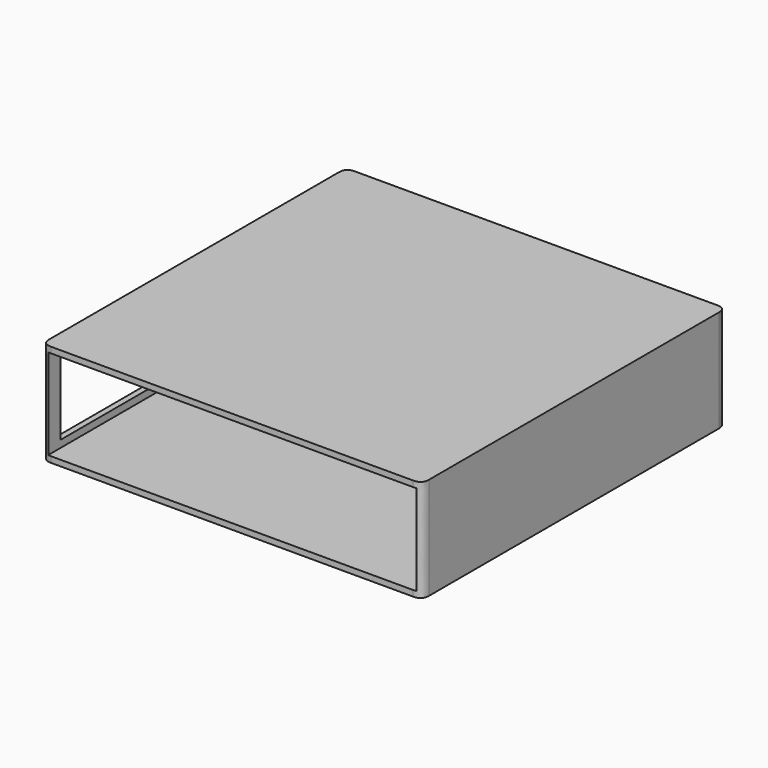
from build123d import *

# Parameters (mm, degrees)
F0_W        = 130
F0_H        = 130
F1_DEPTH    = 17.5
F2_W        = 126
F2_H        = 31
F3_DEPTH    = 126
F5_W        = 122.3782406645
F5_H        = 23.2565429012
F6_DEPTH    = 7
F4_W        = 119.2743226562
F4_H        = 26.0036256061
F7_DEPTH    = 3
F8_T1_DEPTH = 50


# Not quite as in the source:
# - a fillet or chamfer that OpenCascade refuses, or shapes differently, is made with other operations: its cross-section is extruded or revolved along the edge and cut away or added


with BuildPart() as f1:
    # F0 (on Top) → F1 (new body, symmetric)
    with BuildSketch(Plane.XY):
        with Locations((2.0031377077, 1.1643140912)):
            Rectangle(F0_W, F0_H)
    extrude(amount=F1_DEPTH, both=True)

    # F2 (on face) → F3 (cut)
    with BuildSketch(Plane.XZ.offset(63.8356859088)):
        with Locations((2.0031377077, 0)):
            Rectangle(F2_W, F2_H)
    extrude(amount=-F3_DEPTH, mode=Mode.SUBTRACT)

    # F5 (on face) → F6 (cut)
    with BuildSketch(Plane(origin=(0, 66.1643140912, 0), x_dir=(-1, 0, 0), z_dir=(0, 1, 0))):
        with Locations((-2.0031377077, 0)):
            Rectangle(F5_W, F5_H)
    extrude(amount=-F6_DEPTH, mode=Mode.SUBTRACT)

    # F4 (on face) → F7 (cut)
    with BuildSketch(Plane(origin=(-62.9968622923, 0, 0), x_dir=(0, -1, 0), z_dir=(-1, 0, 0))):
        with Locations((-1.2152138836, -0.0606838628)):
            Rectangle(F4_W, F4_H)
    extrude(amount=-F7_DEPTH, mode=Mode.SUBTRACT)

    # F8: fillet of radius 3 on 4 edges, made by hand

    # F8_s2 → F8_t1 (cut)
    with BuildSketch(Plane.XY.offset(-25)):
        with BuildLine():
            add(Edge.make_bspline(
                [(-59.9968622923, 66.1643140912), (-62.9968622923, 66.1643140912), (-62.9968622923, 63.1643140912)],
                knots=[0, 0, 0, 1, 1, 1], degree=2, weights=[1, 1, 1]))
            Line((-62.9968622923, 63.1643140912), (-62.9968622923, 66.1643140912))
            Line((-62.9968622923, 66.1643140912), (-59.9968622923, 66.1643140912))
        make_face()
        with BuildLine():
            add(Edge.make_bspline(
                [(-62.9968622923, -60.8356859088), (-62.9968622923, -63.8356859088), (-59.9968622923, -63.8356859088)],
                knots=[0, 0, 0, 1, 1, 1], degree=2, weights=[1, 1, 1]))
            Line((-59.9968622923, -63.8356859088), (-62.9968622923, -63.8356859088))
            Line((-62.9968622923, -63.8356859088), (-62.9968622923, -60.8356859088))
        make_face()
        with BuildLine():
            add(Edge.make_bspline(
                [(64.0031377077, 66.1643140912), (67.0031377077, 66.1643140912), (67.0031377077, 63.1643140912)],
                knots=[0, 0, 0, 1, 1, 1], degree=2, weights=[1, 1, 1]))
            Line((67.0031377077, 63.1643140912), (67.0031377077, 66.1643140912))
            Line((67.0031377077, 66.1643140912), (64.0031377077, 66.1643140912))
        make_face()
        with BuildLine():
            add(Edge.make_bspline(
                [(67.0031377077, -60.8356859088), (67.0031377077, -63.8356859088), (64.0031377077, -63.8356859088)],
                knots=[0, 0, 0, 1, 1, 1], degree=2, weights=[1, 1, 1]))
            Line((64.0031377077, -63.8356859088), (67.0031377077, -63.8356859088))
            Line((67.0031377077, -63.8356859088), (67.0031377077, -60.8356859088))
        make_face()
    extrude(amount=F8_T1_DEPTH, mode=Mode.SUBTRACT)


solid = f1.part
